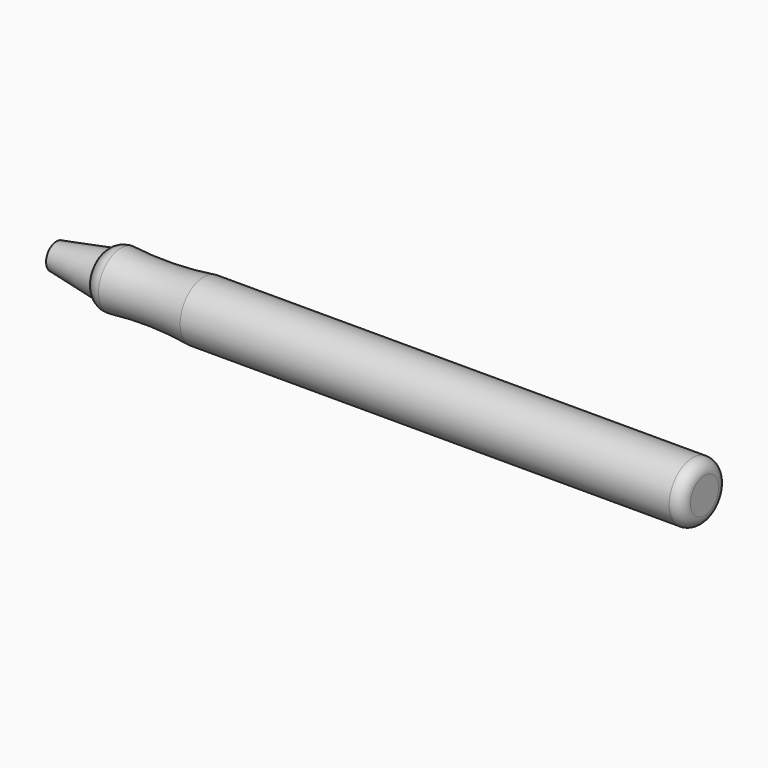
from build123d import *

# Parameters (mm, degrees)
F2_R     = 2.54
F3_R     = 2.159
F4_DEPTH = 127


# Not quite as in the source:
# - a fillet or chamfer that OpenCascade refuses, or shapes differently, is made with other operations: its cross-section is extruded or revolved along the edge and cut away or added


with BuildPart() as f1:
    # F0 (on Top) → F1 (revolve)
    with BuildSketch(Plane.XY):
        with BuildLine():
            Line((0, 2.794), (0, 0))
            Line((0, 0), (139.7, 0))
            Line((139.7, 0), (139.7, 6.35))
            Line((139.7, 6.35), (31.75, 6.35))
            ThreePointArc((31.75, 6.35), (21.3842908829, 5.6416689079), (11.0185817658, 6.35))
            ThreePointArc((11.0185817658, 6.35), (10.9918000406, 5.5558048596), (11.0379582651, 4.7625))
            Line((11.0379582651, 4.7625), (0, 2.794))
        make_face()
    revolve(axis=Axis((69.85, 0, 0), (1, 0, 0)))

    # F2
    f2_edges = [f1.edges().sort_by_distance(p)[0] for p in [
        (139.7, -6.35, 0),
    ]]
    fillet(f2_edges, radius=F2_R)

    # F3 (on face) → F4 (cut)
    with BuildSketch(Plane(origin=(0, 0, 0), x_dir=(0, -1, 0), z_dir=(-1, 0, 0))):
        Circle(F3_R)
    extrude(amount=-F4_DEPTH, mode=Mode.SUBTRACT)

    # F5: fillet of radius 3.175 on 1 edges, made by hand

    # F5_s1 → F5_t2 (revolve, cut)
    with BuildSketch(Plane.XY):
        with BuildLine():
            ThreePointArc((13.886159803, 6.0114768317), (12.2986630958, 5.7596010622), (11.0379582651, 4.7625))
            Line((11.0379582651, 4.7625), (10.9872426769, 4.8007122901))
            ThreePointArc((10.9872426769, 4.8007122901), (10.9283047702, 5.5550298573), (10.9552829498, 6.3550507327))
            Line((10.9552829498, 6.3550507327), (11.0272198567, 6.4129097241))
            ThreePointArc((11.0272198567, 6.4129097241), (12.4582117618, 6.2302164435), (13.8924082455, 6.0746686585))
            Line((13.8924082455, 6.0746686585), (13.886159803, 6.0114768317))
        make_face()
    revolve(axis=Axis((11.0185817658, 0, 0), (1, 0, 0)), mode=Mode.SUBTRACT)


solid = f1.part
